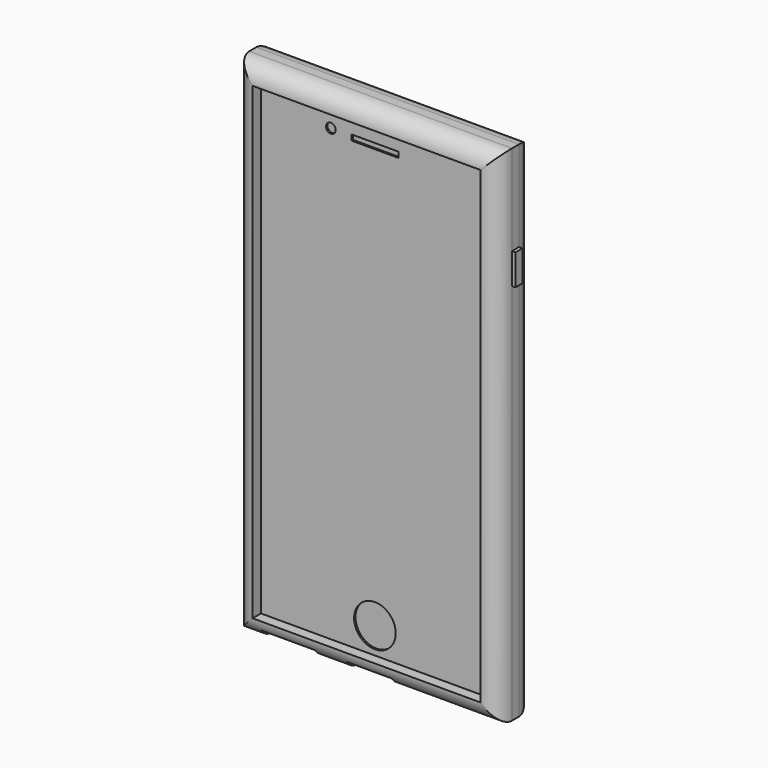
from build123d import *

# Parameters (mm, degrees)
F0_W      = 76.2
F0_H      = 146.05
F1_DEPTH  = 12.7
F2_R      = 5.08
F3_R      = 5.08
F4_DEPTH  = 2.54
F5_W      = 2.4973305091
F5_H      = 11.7452070117
F5_W_2    = 2.54
F5_W_3    = 2.9405460703
F6_DEPTH  = 2.54
F7_W      = 2.8808997013
F7_H      = 5.0969719887
F8_DEPTH  = 2.032
F9_W      = 1.4404498506
F9_H      = 5.0969719887
F10_DEPTH = 3.048
F11_W     = 2.54
F11_H     = 11.43
F12_DEPTH = 1.016
F13_W     = 2.54
F13_H     = 11.43
F14_DEPTH = 1.016
F16_DEPTH = 0.508
F17_W     = 15.7348513603
F17_H     = 10.4662538506
F17_H_2   = 4.2268524888
F18_DEPTH = 2.286
F19_W     = 18.1282758713
F19_H     = 1.7902922965
F19_H_2   = 2.54
F19_H_3   = 2.6172961119
F20_DEPTH = 2.286
F21_R     = 2.1027824112
F22_DEPTH = 2.286
F24_DEPTH = 1.27
F25_W     = 13.5468328476
F25_H     = 1.6100406647
F4_FACE_W = 66.04
F4_FACE_H = 135.89
F4_FACE_R = 6.0325
F26_DEPTH = 0.508
F27_R     = 1.3953400064
F28_DEPTH = 0.508
F30_DEPTH = 0.508
F31_W     = 6.604
F31_H     = 3.0624943002
F31_H_2   = 5.8275056998
F31_H_3   = 2.54
F32_DEPTH = 2.286
F34_DEPTH = 1.27
F35_W     = 24.4420864832
F35_H     = 11.2134301376
F36_DEPTH = 2.286
F39_R     = 2.3136513578
F40_DEPTH = 0.254
F42_DEPTH = 1.016
F43_DEPTH = 1.778
F44_W     = 2.54
F44_H     = 8.934661746
F45_DEPTH = 1.016


# Not quite as in the source:
# - the program builds the solid bodies; features that only make, move or delete a surface that nothing else refers to are left out


with BuildPart() as f1:
    # F0 (on Front) → F1 (new body)
    with BuildSketch(Plane.XZ):
        with Locations((38.1, 73.025)):
            Rectangle(F0_W, F0_H)
    extrude(amount=F1_DEPTH)

    # F2
    f2_edges = [f1.edges().sort_by_distance(p)[0] for p in [
        (0, -12.7, 73.025),
        (38.1, -12.7, 0),
        (76.2, -12.7, 73.025),
        (38.1, -12.7, 146.05),
    ]]
    fillet(f2_edges, radius=F2_R)

    # F3
    f3_edges = [f1.edges().sort_by_distance(p)[0] for p in [
        (0, 0, 73.025),
        (38.1, 0, 0),
        (76.2, 0, 73.025),
        (38.1, 0, 146.05),
    ]]
    fillet(f3_edges, radius=F3_R)

    # F4 (cut): a face of the model
    f4_faces = [f1.faces().sort_by_distance(p)[0] for p in [
        (38.1, -12.7, 73.025),
    ]]
    extrude(f4_faces, amount=-F4_DEPTH, mode=Mode.SUBTRACT)

    # F5 (on face) → F6 (cut)
    with BuildSketch(Plane(origin=(0, 0, 0), x_dir=(0, -1, 0), z_dir=(-1, 0, 0))):
        with Locations((3.8313347455, 127.8729029)):
            Rectangle(F5_W, F5_H)
        with Locations((6.35, 127.8729029)):
            Rectangle(F5_W_2, F5_H)
        with Locations((9.0902730352, 127.8729029)):
            Rectangle(F5_W_3, F5_H)
    extrude(amount=-F6_DEPTH, mode=Mode.SUBTRACT)

    # F7 (on face) → F8 (join)
    with BuildSketch(Plane(origin=(2.54, 0, 0), x_dir=(0, -1, 0), z_dir=(-1, 0, 0))):
        with Locations((6.2391965184, 127.6512891054)):
            Rectangle(F7_W, F7_H)
    extrude(amount=F8_DEPTH)

    # F9 (on face) → F10 (cut)
    with BuildSketch(Plane(origin=(0.508, 0, 0), x_dir=(0, -1, 0), z_dir=(-1, 0, 0))):
        with Locations((6.9594214438, 127.6512891054)):
            Rectangle(F9_W, F9_H)
    extrude(amount=-F10_DEPTH, mode=Mode.SUBTRACT)

    # F11 (on face) → F12 (join)
    with BuildSketch(Plane(origin=(0, 0, 0), x_dir=(0, -1, 0), z_dir=(-1, 0, 0))):
        with Locations((6.35, 112.3141669893)):
            Rectangle(F11_W, F11_H)
    extrude(amount=F12_DEPTH)

    # F13 (on face) → F14 (join)
    with BuildSketch(Plane(origin=(0, 0, 0), x_dir=(0, -1, 0), z_dir=(-1, 0, 0))):
        with Locations((6.35, 97.9860373998)):
            Rectangle(F13_W, F13_H)
    extrude(amount=F14_DEPTH)

    # F15 (on face) → F16 (cut)
    with BuildSketch(Plane.XZ.offset(10.16)):
        with BuildLine():
            ThreePointArc((44.1325, 12.7), (33.8343783425, 16.9656216575), (38.1, 6.6675))
            ThreePointArc((38.1, 6.6675), (42.3656216575, 8.4343783425), (44.1325, 12.7))
        make_face()
    extrude(amount=-F16_DEPTH, mode=Mode.SUBTRACT)

    # F17 (on face) → F18 (cut)
    with BuildSketch(Plane(origin=(0, 0, 0), x_dir=(1, 0, 0), z_dir=(0, 0, -1))):
        with Locations((14.6331973374, 6.6137255635)):
            Rectangle(F17_W, F17_H)
        with Locations((14.6331973374, 9.7334262444)):
            Rectangle(F17_W, F17_H_2)
    extrude(amount=-F18_DEPTH, mode=Mode.SUBTRACT)

    # F19 (on face) → F20 (cut)
    with BuildSketch(Plane(origin=(0, 0, 0), x_dir=(1, 0, 0), z_dir=(0, 0, -1))):
        with Locations((61.1127465963, 4.1848538518)):
            Rectangle(F19_W, F19_H)
        with Locations((61.1127465963, 6.35)):
            Rectangle(F19_W, F19_H_2)
        with Locations((61.1127465963, 8.9286480559)):
            Rectangle(F19_W, F19_H_3)
    extrude(amount=-F20_DEPTH, mode=Mode.SUBTRACT)

    # F21 (on face) → F22 (cut)
    with BuildSketch(Plane(origin=(0, 0, 2.286), x_dir=(1, 0, 0), z_dir=(0, 0, -1))):
        with Locations((14.4449183717, 6.7520015873)):
            Circle(F21_R)
    extrude(amount=-F22_DEPTH, mode=Mode.SUBTRACT)

    # F23 (on face) → F24 (cut)
    with BuildSketch(Plane(origin=(0, 0, 2.286), x_dir=(1, 0, 0), z_dir=(0, 0, -1))):
        with BuildLine():
            ThreePointArc((54.0211938972, 6.1539337039), (53.2591938972, 6.9159337039), (52.4971938972, 6.1539337039))
            Line((52.4971938972, 6.1539337039), (54.0211938972, 6.1539337039))
        make_face()
        with BuildLine():
            ThreePointArc((69.8944770451, 6.1539337039), (69.1324770451, 6.9159337039), (68.3704770451, 6.1539337039))
            Line((68.3704770451, 6.1539337039), (69.8944770451, 6.1539337039))
        make_face()
        with BuildLine():
            Line((69.8944770451, 6.1539337039), (68.3704770451, 6.1539337039))
            ThreePointArc((68.3704770451, 6.1539337039), (69.1324770451, 5.3919337039), (69.8944770451, 6.1539337039))
        make_face()
        with BuildLine():
            ThreePointArc((67.8202428575, 6.1539337039), (67.0582428575, 6.9159337039), (66.2962428575, 6.1539337039))
            Line((66.2962428575, 6.1539337039), (67.8202428575, 6.1539337039))
        make_face()
        with BuildLine():
            Line((67.8202428575, 6.1539337039), (66.2962428575, 6.1539337039))
            ThreePointArc((66.2962428575, 6.1539337039), (67.0582428575, 5.3919337039), (67.8202428575, 6.1539337039))
        make_face()
        with BuildLine():
            ThreePointArc((65.8047863002, 6.1539337039), (65.0427863002, 6.9159337039), (64.2807863002, 6.1539337039))
            Line((64.2807863002, 6.1539337039), (65.8047863002, 6.1539337039))
        make_face()
        with BuildLine():
            Line((65.8047863002, 6.1539337039), (64.2807863002, 6.1539337039))
            ThreePointArc((64.2807863002, 6.1539337039), (65.0427863002, 5.3919337039), (65.8047863002, 6.1539337039))
        make_face()
        with BuildLine():
            ThreePointArc((63.588320529, 6.1539337039), (62.826320529, 6.9159337039), (62.064320529, 6.1539337039))
            Line((62.064320529, 6.1539337039), (63.588320529, 6.1539337039))
        make_face()
        with BuildLine():
            Line((63.588320529, 6.1539337039), (62.064320529, 6.1539337039))
            ThreePointArc((62.064320529, 6.1539337039), (62.826320529, 5.3919337039), (63.588320529, 6.1539337039))
        make_face()
        with BuildLine():
            ThreePointArc((61.1659095342, 6.1539337039), (60.4039095342, 6.9159337039), (59.6419095342, 6.1539337039))
            Line((59.6419095342, 6.1539337039), (61.1659095342, 6.1539337039))
        make_face()
        with BuildLine():
            Line((61.1659095342, 6.1539337039), (59.6419095342, 6.1539337039))
            ThreePointArc((59.6419095342, 6.1539337039), (60.4039095342, 5.3919337039), (61.1659095342, 6.1539337039))
        make_face()
        with BuildLine():
            ThreePointArc((58.6699277813, 6.1539337039), (57.9079277813, 6.9159337039), (57.1459277813, 6.1539337039))
            Line((57.1459277813, 6.1539337039), (58.6699277813, 6.1539337039))
        make_face()
        with BuildLine():
            Line((58.6699277813, 6.1539337039), (57.1459277813, 6.1539337039))
            ThreePointArc((57.1459277813, 6.1539337039), (57.9079277813, 5.3919337039), (58.6699277813, 6.1539337039))
        make_face()
        with BuildLine():
            ThreePointArc((56.3848160858, 6.1539337039), (55.6228160858, 6.9159337039), (54.8608160858, 6.1539337039))
            Line((54.8608160858, 6.1539337039), (56.3848160858, 6.1539337039))
        make_face()
        with BuildLine():
            Line((56.3848160858, 6.1539337039), (54.8608160858, 6.1539337039))
            ThreePointArc((54.8608160858, 6.1539337039), (55.6228160858, 5.3919337039), (56.3848160858, 6.1539337039))
        make_face()
        with BuildLine():
            Line((54.0211938972, 6.1539337039), (52.4971938972, 6.1539337039))
            ThreePointArc((52.4971938972, 6.1539337039), (53.2591938972, 5.3919337039), (54.0211938972, 6.1539337039))
        make_face()
    extrude(amount=-F24_DEPTH, mode=Mode.SUBTRACT)

    # F25 (on face) + F4_face (on face) → F26 (cut)
    with BuildSketch(Plane.XZ.offset(9.652)):
        with Locations((38.1, 135.0751519203)):
            Rectangle(F25_W, F25_H)
    with BuildSketch(Plane(origin=(38.1, -10.16, 73.025), x_dir=(1, 0, 0), z_dir=(0, -1, 0))):
        Rectangle(F4_FACE_W, F4_FACE_H)
        with Locations((0, -60.325)):
            Circle(F4_FACE_R, mode=Mode.SUBTRACT)
    extrude(amount=-F26_DEPTH, mode=Mode.SUBTRACT)

    # F27 (on face) → F28 (cut)
    with BuildSketch(Plane.XZ.offset(9.652)):
        with Locations((25.323253125, 135.4901641607)):
            Circle(F27_R)
    extrude(amount=-F28_DEPTH, mode=Mode.SUBTRACT)

    # F29 (on face) → F30 (cut)
    with BuildSketch(Plane.XZ.offset(9.652)):
        with BuildLine():
            ThreePointArc((44.1325, 12.7), (33.8343783425, 16.9656216575), (38.1, 6.6675))
            ThreePointArc((38.1, 6.6675), (42.3656216575, 8.4343783425), (44.1325, 12.7))
        make_face()
    extrude(amount=-F30_DEPTH, mode=Mode.SUBTRACT)

    # F31 (on face) → F32 (cut)
    with BuildSketch(Plane(origin=(0, 0, 0), x_dir=(1, 0, 0), z_dir=(0, 0, -1))):
        with Locations((34.9296401281, 3.5487528499)):
            Rectangle(F31_W, F31_H)
        with Locations((41.5336401281, 10.5337528499)):
            Rectangle(F31_W, F31_H_2)
        with Locations((41.5336401281, 3.5487528499)):
            Rectangle(F31_W, F31_H)
        with Locations((34.9296401281, 6.35)):
            Rectangle(F31_W, F31_H_3)
        with Locations((41.5336401281, 6.35)):
            Rectangle(F31_W, F31_H_3)
        with Locations((34.9296401281, 10.5337528499)):
            Rectangle(F31_W, F31_H_2)
    extrude(amount=-F32_DEPTH, mode=Mode.SUBTRACT)

    # F33 (on face) → F34 (cut)
    with BuildSketch(Plane(origin=(0, 0, 2.286), x_dir=(1, 0, 0), z_dir=(0, 0, -1))):
        Polygon((34.6526485043, 7.9915548147), (34.6526485043, 6.9400710721), (34.6526485043, 5.8885873295), (41.810631752, 5.8885873295), (41.810631752, 7.9915548147), align=None)
    extrude(amount=-F34_DEPTH, mode=Mode.SUBTRACT)

    # F35 (on face) → F36 (cut)
    with BuildSketch(Plane(origin=(0, 0, 0), x_dir=(-1, 0, 0), z_dir=(0, 1, 0))):
        with Locations((-58.8989567584, 135.3632849312)):
            Rectangle(F35_W, F35_H)
    extrude(amount=-F36_DEPTH, mode=Mode.SUBTRACT)

    # F39 (on face) → F40 (cut)
    with BuildSketch(Plane(origin=(0, -2.286, 0), x_dir=(-1, 0, 0), z_dir=(0, 1, 0))):
        with Locations((-53.6911524832, 134.4103217125)):
            Circle(F39_R)
    extrude(amount=-F40_DEPTH, mode=Mode.SUBTRACT)

    # F41 (on face) → F42 (cut)
    with BuildSketch(Plane(origin=(0, 0, 0), x_dir=(-1, 0, 0), z_dir=(0, 1, 0))):
        with BuildLine():
            ThreePointArc((-38.1, 122.8167432735), (-46.1358037085, 103.4165969759), (-26.7356574109, 111.4524006844))
            ThreePointArc((-26.7356574109, 111.4524006844), (-30.0641962915, 119.4882043929), (-38.1, 122.8167432735))
        make_face()
        with BuildLine():
            ThreePointArc((-26.7356574109, 111.4524006844), (-30.0641962915, 119.4882043929), (-38.1, 122.8167432735))
            ThreePointArc((-38.1, 122.8167432735), (-46.1358037085, 103.4165969759), (-26.7356574109, 111.4524006844))
        make_face()
    extrude(amount=-F42_DEPTH, mode=Mode.SUBTRACT)

    # F43 (cut): a face of the model
    f43_faces = [f1.faces().sort_by_distance(p)[0] for p in [
        (38.1, -1.016, 111.4524006844),
    ]]
    extrude(f43_faces, amount=-F43_DEPTH, mode=Mode.SUBTRACT)

    # F44 (on face) → F45 (join)
    with BuildSketch(Plane.YZ.offset(76.2)):
        with Locations((-6.35, 115.3773292899)):
            Rectangle(F44_W, F44_H)
    extrude(amount=F45_DEPTH)


solid = f1.part
